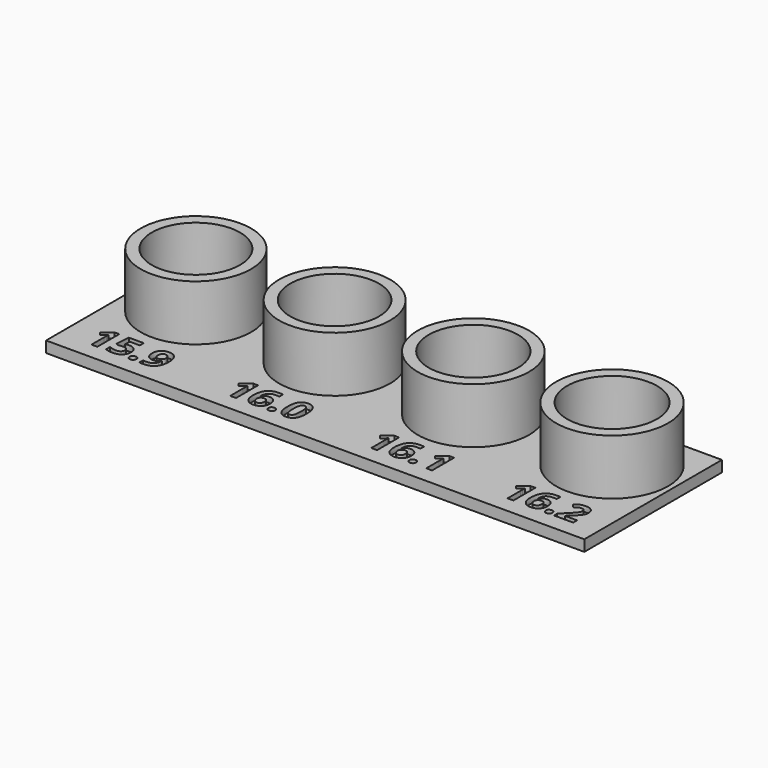
from build123d import *

# Parameters (mm, degrees)
F0_R         = 9.95
F0_R_2       = 7.95
F1_DEPTH     = 10
F0_R_3       = 10
F0_R_4       = 8
F0_R_5       = 10.05
F0_R_6       = 8.05
F0_R_7       = 10.1
F0_R_8       = 8.1
F2_W         = 97
F2_H         = 31
F3_DEPTH     = 2
F5_TEXT_SIZE = 6.9444444444
F6_DEPTH     = 1


# Not quite as in the source:
# - Text() gives the source's letters only with a copy of the font that has no kerning and outlines rounded to 1/6400 em; it was checked with that copy


with BuildPart() as f1:
    # F0 (on Top) → F1 (new body)
    with BuildSketch(Plane.XY):
        with Locations((-75, 0)):
            Circle(F0_R)
        with Locations((-75, 0)):
            Circle(F0_R_2, mode=Mode.SUBTRACT)
    extrude(amount=F1_DEPTH)


with BuildPart() as f1b:
    # F0 (on Top) → F1, piece 2 (new body)
    with BuildSketch(Plane.XY):
        with Locations((-50, 0)):
            Circle(F0_R_3)
        with Locations((-50, 0)):
            Circle(F0_R_4, mode=Mode.SUBTRACT)
    extrude(amount=F1_DEPTH)


with BuildPart() as f1c:
    # F0 (on Top) → F1, piece 3 (new body)
    with BuildSketch(Plane.XY):
        with Locations((-25, 0)):
            Circle(F0_R_5)
        with Locations((-25, 0)):
            Circle(F0_R_6, mode=Mode.SUBTRACT)
    extrude(amount=F1_DEPTH)


with BuildPart() as f1d:
    # F0 (on Top) → F1, piece 4 (new body)
    with BuildSketch(Plane.XY):
        Circle(F0_R_7)
        Circle(F0_R_8, mode=Mode.SUBTRACT)
    extrude(amount=F1_DEPTH)


with BuildPart() as f3:
    # F2 (on Top) → F3 (new body)
    with BuildSketch(Plane.XY):
        with Locations((-37.5, -4.5)):
            Rectangle(F2_W, F2_H)
    extrude(amount=-F3_DEPTH)


with BuildPart() as f1_1:
    add(f1.part)

    # F4: union F1b, F1c, F1d, F3
    add(f1b.part)
    add(f1c.part)
    add(f1d.part)
    add(f3.part)

    # F5 (on face) → F6 (cut)
    with BuildSketch(Plane.XY):
        with Locations((-31.6134982639, -17.0000005421)):
            Text('16.1', F5_TEXT_SIZE, font='Open Sans', font_style=FontStyle.BOLD, text_align=(TextAlign.LEFT, TextAlign.BOTTOM))
        with Locations((-7.05078125, -17)):
            Text('16.2', F5_TEXT_SIZE, font='Open Sans', font_style=FontStyle.BOLD, text_align=(TextAlign.LEFT, TextAlign.BOTTOM))
        with Locations((-82.0404730903, -17)):
            Text('15.9', F5_TEXT_SIZE, font='Open Sans', font_style=FontStyle.BOLD, text_align=(TextAlign.LEFT, TextAlign.BOTTOM))
        with Locations((-57.0372178819, -17)):
            Text('16.0', F5_TEXT_SIZE, font='Open Sans', font_style=FontStyle.BOLD, text_align=(TextAlign.LEFT, TextAlign.BOTTOM))
    extrude(amount=-F6_DEPTH, mode=Mode.SUBTRACT)


solid = f1_1.part
